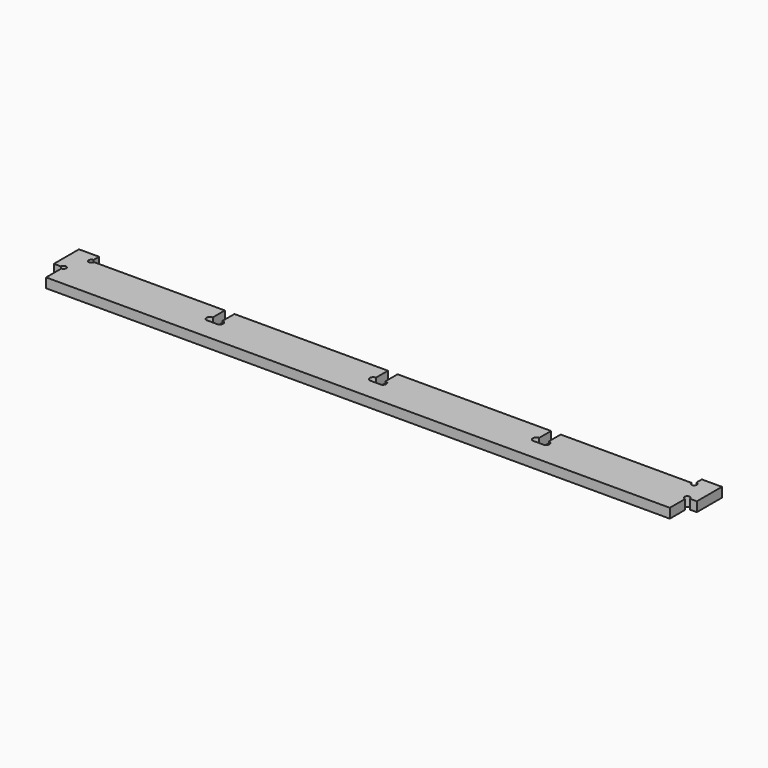
from build123d import *

# Parameters (mm, degrees)
F1_W      = 1219.2
F1_H      = 82.55
F2_DEPTH  = 18.2118
F4_DEPTH  = 18.2128
F6_DEPTH  = 18.2128
F7_W      = 38.1
F7_H      = 18.2118
F8_DEPTH  = 18.2118
F9_R      = 5.08
F10_DEPTH = 18.2128


# Not quite as in the source:
# - a variable given as a bare number and used for a length is read in inches; the dataset says mm whatever the document's units were


with BuildPart() as f2:
    # F1 (on Top) → F2 (new body)
    with BuildSketch(Plane.XY):
        Rectangle(F1_W, F1_H)
    extrude(amount=F2_DEPTH)

    # F3 (on face) → F4 (cut, through all)
    with BuildSketch(Plane.XY.offset(18.2118)):
        Polygon((-609.6, 0), (-609.6, -41.275), (-591.3882, -41.275), (-591.3882, -5.08), (-591.3882, 0), (-596.4682, 0), align=None)
        with BuildLine():
            Line((-591.3882, 0), (-591.3882, -5.08))
            ThreePointArc((-591.3882, -5.08), (-587.7960975516, 3.5921024484), (-596.4682, 0))
            Line((-596.4682, 0), (-591.3882, 0))
        make_face()
        with BuildLine():
            Line((591.3882, 0), (596.4682, 0))
            ThreePointArc((596.4682, 0), (587.7960975516, 3.5921024484), (591.3882, -5.08))
            Line((591.3882, -5.08), (591.3882, 0))
        make_face()
        Polygon((591.3882, -5.08), (591.3882, -41.275), (609.6, -41.275), (609.6, 0), (596.4682, 0), (591.3882, 0), align=None)
    extrude(amount=-F4_DEPTH, mode=Mode.SUBTRACT)

    # F5 (on face) → F6 (cut, through all)
    with BuildSketch(Plane.XY.offset(18.2118)):
        Polygon((-300.24705, 41.275), (-318.45885, 41.275), (-318.45885, 12.954), (-318.45885, 0), (-316.6449271791, 0), (-302.0609728209, 0), (-300.24705, 0), (-300.24705, 12.954), align=None)
        with BuildLine():
            Line((-318.45885, 0), (-318.45885, 12.954))
            ThreePointArc((-318.45885, 12.954), (-324.9990417403, 5.434189976), (-316.6449271791, 0))
            Line((-316.6449271791, 0), (-318.45885, 0))
        make_face()
        with BuildLine():
            ThreePointArc((-302.0609728209, 0), (-293.7068582597, 5.434189976), (-300.24705, 12.954))
            Line((-300.24705, 12.954), (-300.24705, 0))
            Line((-300.24705, 0), (-302.0609728209, 0))
        make_face()
        Polygon((318.45885, 41.275), (300.24705, 41.275), (300.24705, 12.954), (300.24705, 0), (302.0609728208, 0), (316.6449271792, 0), (318.45885, 0), (318.45885, 12.954), align=None)
        with BuildLine():
            Line((300.24705, 0), (300.24705, 12.954))
            ThreePointArc((300.24705, 12.954), (293.7068582597, 5.434189976), (302.0609728208, 0))
            Line((302.0609728208, 0), (300.24705, 0))
        make_face()
        with BuildLine():
            ThreePointArc((316.6449271792, 0), (324.9990417403, 5.434189976), (318.45885, 12.954))
            Line((318.45885, 12.954), (318.45885, 0))
            Line((318.45885, 0), (316.6449271792, 0))
        make_face()
        Polygon((9.1059, 41.275), (-9.1059, 41.275), (-9.1059, 12.954), (-9.1059, 0), (-7.2919771792, 0), (7.2919771792, 0), (9.1059, 0), (9.1059, 12.954), align=None)
        with BuildLine():
            Line((-9.1059, 0), (-9.1059, 12.954))
            ThreePointArc((-9.1059, 12.954), (-15.6460917403, 5.434189976), (-7.2919771792, 0))
            Line((-7.2919771792, 0), (-9.1059, 0))
        make_face()
        with BuildLine():
            ThreePointArc((7.2919771792, 0), (15.6460917403, 5.434189976), (9.1059, 12.954))
            Line((9.1059, 12.954), (9.1059, 0))
            Line((9.1059, 0), (7.2919771792, 0))
        make_face()
    extrude(amount=-F6_DEPTH, mode=Mode.SUBTRACT)

    # F7 (on face) → F8 (join)
    with BuildSketch(Plane(origin=(0, 41.275, 0), x_dir=(-1, 0, 0), z_dir=(0, 1, 0))):
        with Locations((590.55, 9.1059)):
            Rectangle(F7_W, F7_H)
        with Locations((-590.55, 9.1059)):
            Rectangle(F7_W, F7_H)
    extrude(amount=F8_DEPTH)

    # F9 (on face) → F10 (cut, through all)
    with BuildSketch(Plane(origin=(0, 0, 0), x_dir=(1, 0, 0), z_dir=(0, 0, -1))):
        with Locations((571.5, -41.275)):
            Circle(F9_R)
        with Locations((-571.5, -41.275)):
            Circle(F9_R)
    extrude(amount=-F10_DEPTH, mode=Mode.SUBTRACT)


solid = f2.part
